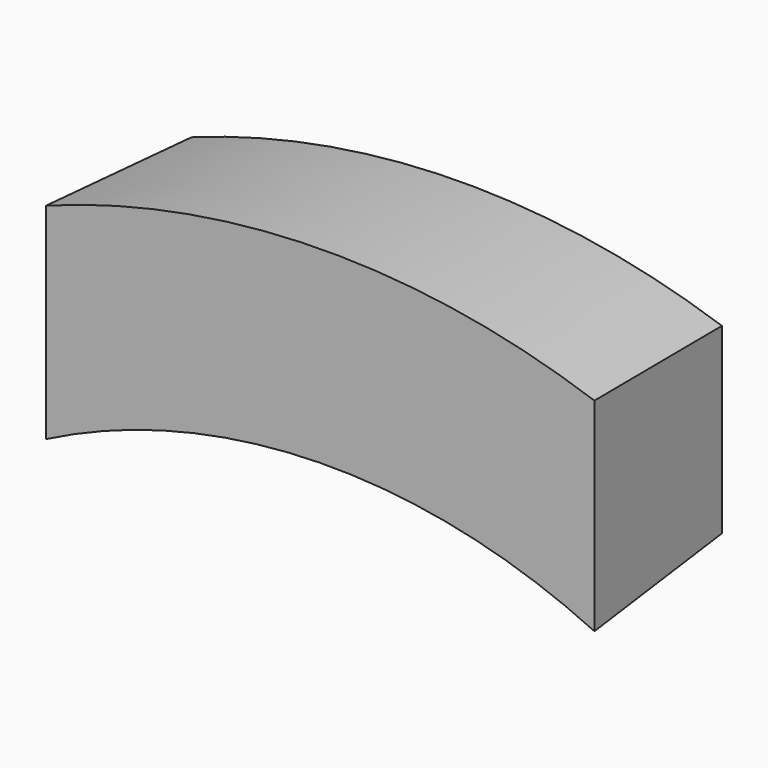
from build123d import *

# Parameters (mm, degrees)
F1_DEPTH               = 25.4
DRAFT_F1_DRAFTED_ANGLE = -3


# Not quite as in the source:
# - an extrude with a draft is written as a straight extrude whose walls are then drafted


with BuildPart() as f1:
    # F0 (on Front) → F1 (new body)
    with BuildSketch(Plane.XZ):
        with BuildLine():
            ThreePointArc((18.6881478876, 52.4278291636), (-20.9018950369, 58.6626133257), (-60.3266693652, 51.4562826731))
            Line((-60.3266693652, 51.4562826731), (-60.3266693652, 23.9205155522))
            ThreePointArc((-60.3266693652, 23.9205155522), (-20.9604910306, 33.259241705), (18.6881478876, 25.2036079764))
            Line((18.6881478876, 25.2036079764), (18.6881478876, 52.4278291636))
        make_face()
    extrude(amount=F1_DEPTH)

    # draft_F1_drafted
    draft_f1_drafted_walls = [f1.faces().sort_by_distance(p)[0] for p in [
        (18.6881478876, -16.9333333333, 38.81571857),
        (-20.9018950369, -16.9333333333, 58.6626133257),
        (-60.3266693652, -16.9333333333, 37.6883991126),
        (-20.9604910306, -16.9333333333, 33.259241705),
    ]]
    draft(draft_f1_drafted_walls, neutral_plane=Plane.XZ, angle=DRAFT_F1_DRAFTED_ANGLE)


solid = f1.part
